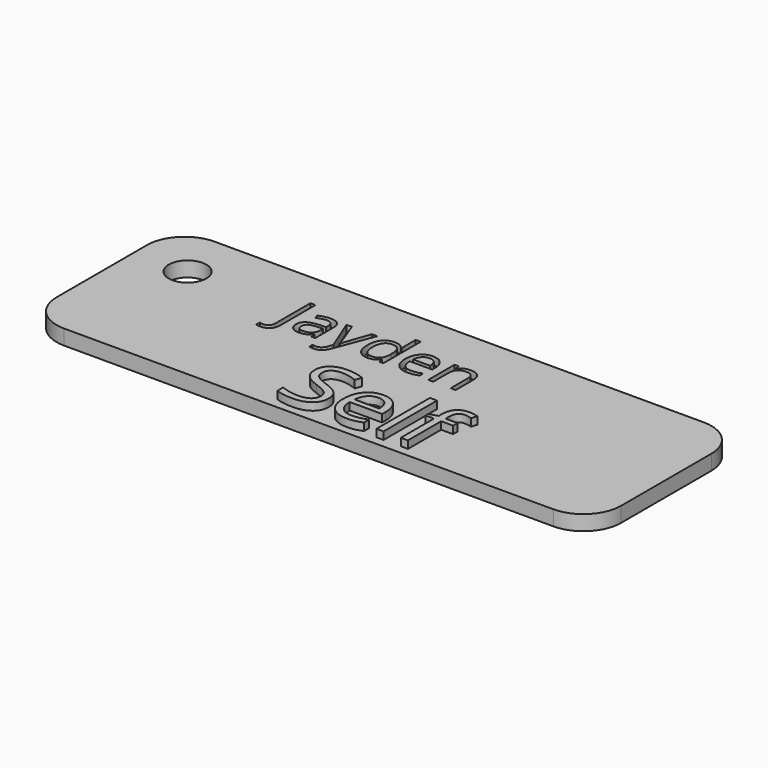
from build123d import *

# Parameters (mm, degrees)
F1_DEPTH     = 2
F3_D         = 5
F4_TEXT_SIZE = 8.1449168243
F5_DEPTH     = 1
F6_TEXT_SIZE = 11.6769382859
F7_DEPTH     = 1


# Not quite as in the source:
# - Text() gives the source's letters only with a copy of the font that has no kerning and outlines rounded to 1/6400 em; it was checked with that copy


with BuildPart() as f1:
    # F0 (on Top) → F1 (new body)
    with BuildSketch(Plane.XY):
        with BuildLine():
            Line((32.5, 12.5), (-32.5, 12.5))
            ThreePointArc((-32.5, 12.5), (-36.0355339059, 11.0355339059), (-37.5, 7.5))
            Line((-37.5, 7.5), (-37.5, -7.5))
            ThreePointArc((-37.5, -7.5), (-36.0355339059, -11.0355339059), (-32.5, -12.5))
            Line((-32.5, -12.5), (32.5, -12.5))
            ThreePointArc((32.5, -12.5), (36.0355339059, -11.0355339059), (37.5, -7.5))
            Line((37.5, -7.5), (37.5, 7.5))
            ThreePointArc((37.5, 7.5), (36.0355339059, 11.0355339059), (32.5, 12.5))
        make_face()
    extrude(amount=F1_DEPTH)

    # F3 (through all)
    with Locations(Plane.XY.offset(2)):
        with Locations((-30.5, 5.5)):
            Hole(F3_D / 2)

    # F4 (on face) → F5 (cut)
    with BuildSketch(Plane.XY.offset(2)):
        with Locations((-16.863329336, 2.0951449405)):
            Text('Jayden', F4_TEXT_SIZE, font='Open Sans', text_align=(TextAlign.LEFT, TextAlign.BOTTOM))
    extrude(amount=-F5_DEPTH, mode=Mode.SUBTRACT)

    # F6 (on face) → F7 (join)
    with BuildSketch(Plane.XY.offset(2)):
        with Locations((-5.8921216987, -11.3392276689)):
            Text('Self', F6_TEXT_SIZE, font='Open Sans', text_align=(TextAlign.LEFT, TextAlign.BOTTOM))
    extrude(amount=F7_DEPTH)


solid = f1.part
